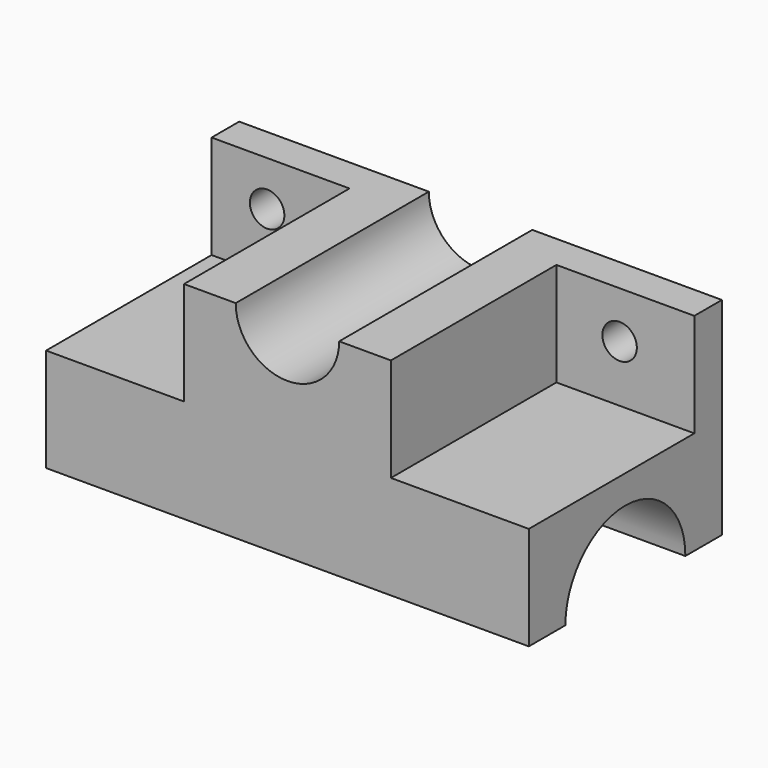
from build123d import *

# Parameters (mm, degrees)
F1_DEPTH = 70
F2_W     = 30
F2_H     = 30
F3_DEPTH = 60
F4_R     = 15
F5_DEPTH = 72.5
F6_R     = 5
F7_DEPTH = 37.8
F8_R     = 5
F9_DEPTH = 25


# Not quite as in the source:
# - a pattern or mirror of a feature is missing from the dataset's text; its kind, count and spacing are read off the source's solid


with BuildPart() as f1:
    # F0 (on Right) → F1 (new body, symmetric)
    with BuildSketch(Plane.YZ):
        with BuildLine():
            Line((10, 30), (0, 30))
            Line((0, 30), (0, 0))
            Line((0, 0), (-60, 0))
            Line((-60, 0), (-60, -30))
            Line((-60, -30), (-46.7469906007, -30))
            ThreePointArc((-46.7469906007, -30), (-25, -8.2530093993), (-3.2530093993, -30))
            Line((-3.2530093993, -30), (10, -30))
            Line((10, -30), (10, 30))
        make_face()
    extrude(amount=F1_DEPTH, both=True)

    # F2 (on face) → F3 (join, through all)
    with BuildSketch(Plane.XZ):
        with Locations((15, 15)):
            Rectangle(F2_W, F2_H)
    f3 = extrude(amount=F3_DEPTH)

    # F3_copies: F3 across plane
    add(f3.mirror(Plane(origin=(0, 0, 0), x_dir=(0, 0, -1), z_dir=(-1, 0, 0))))

    # F4 (on face) → F5 (cut)
    with BuildSketch(Plane.XZ.offset(60)):
        with Locations((0, 30)):
            Circle(F4_R)
    extrude(amount=-F5_DEPTH, mode=Mode.SUBTRACT)

    # F6 (on face) → F7 (cut)
    with BuildSketch(Plane.XZ):
        with Locations((48.3254604042, 16.4307225496)):
            Circle(F6_R)
    extrude(amount=-F7_DEPTH, mode=Mode.SUBTRACT)

    # F8 (on face) → F9 (cut)
    with BuildSketch(Plane.XZ):
        with Locations((-53.8972392678, 16.9797260314)):
            Circle(F8_R)
    extrude(amount=-F9_DEPTH, mode=Mode.SUBTRACT)


solid = f1.part
